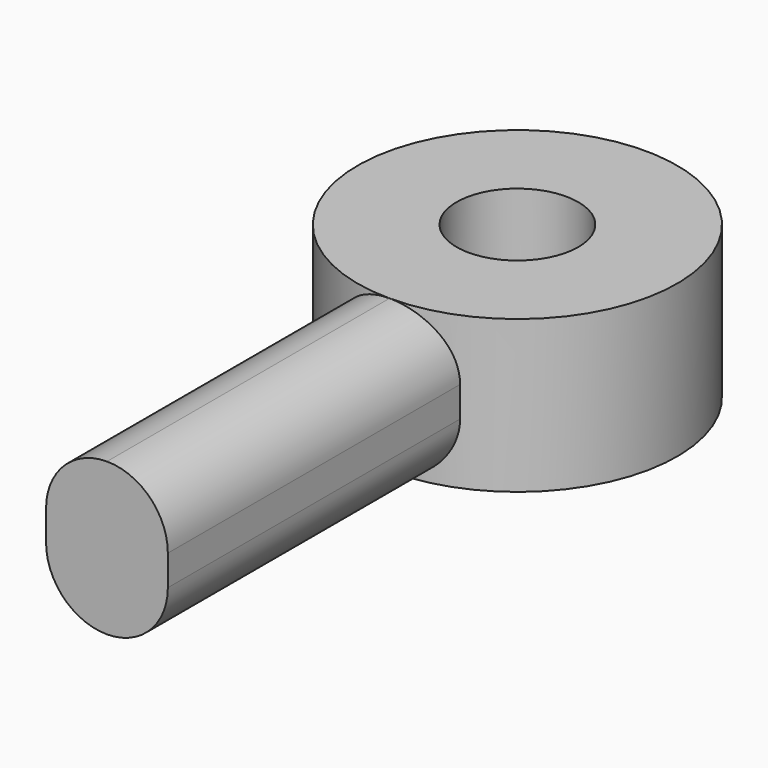
from build123d import *

# Parameters (mm, degrees)
F1_R     = 6.35
F2_DEPTH = 7.9375
F3_R     = 6.34999


# Not quite as in the source:
# - a fillet or chamfer is up to 0.001 mm smaller than in the source, because OpenCascade refuses the exact size


with BuildPart() as f2:
    # F1 (on Top) → F2 (new body, symmetric)
    with BuildSketch(Plane.XY):
        with BuildLine():
            ThreePointArc((6.35, -15.4118372222), (0, 16.66875), (-6.35, -15.4118372222))
            Line((-6.35, -15.4118372222), (-6.35, -53.5118372222))
            Line((-6.35, -53.5118372222), (6.35, -53.5118372222))
            Line((6.35, -53.5118372222), (6.35, -15.4118372222))
        make_face()
        Circle(F1_R, mode=Mode.SUBTRACT)
    extrude(amount=F2_DEPTH, both=True)

    # F3 (radius 6.35 in the source; OpenCascade refuses exactly that, so slightly less here)
    f3_edges = [f2.edges().sort_by_distance(p)[0] for p in [
        (-6.35, -34.461837, -7.9375),
        (6.35, -34.461837, -7.9375),
        (-6.35, -34.461837, 7.9375),
        (6.35, -34.461837, 7.9375),
    ]]
    fillet(f3_edges, radius=F3_R)


solid = f2.part
